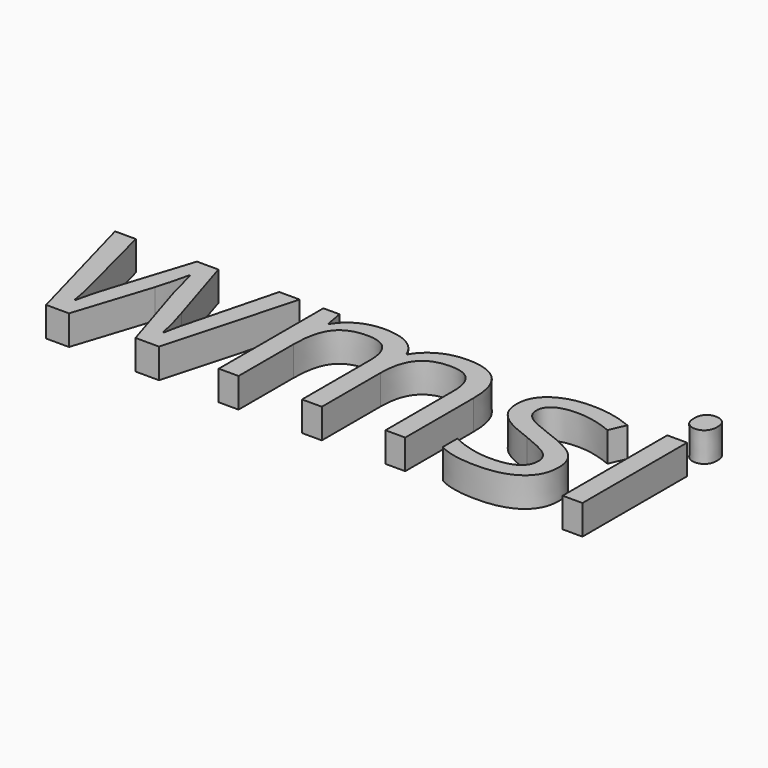
from build123d import *

# Parameters (mm, degrees)
F0_TEXT_SIZE = 20.9511534992
F1_DEPTH     = 2.54


# Not quite as in the source:
# - Text() gives the source's letters only with a copy of the font that has no kerning and outlines rounded to 1/6400 em; it was checked with that copy


with BuildPart() as f1:
    # F0 (on Top) → F1 (new body)
    with BuildSketch(Plane.XY):
        with Locations((-50.8, 0)):
            Text('wmsi', F0_TEXT_SIZE, font='Open Sans', text_align=(TextAlign.LEFT, TextAlign.BOTTOM))
    extrude(amount=F1_DEPTH)


solid = f1.part
